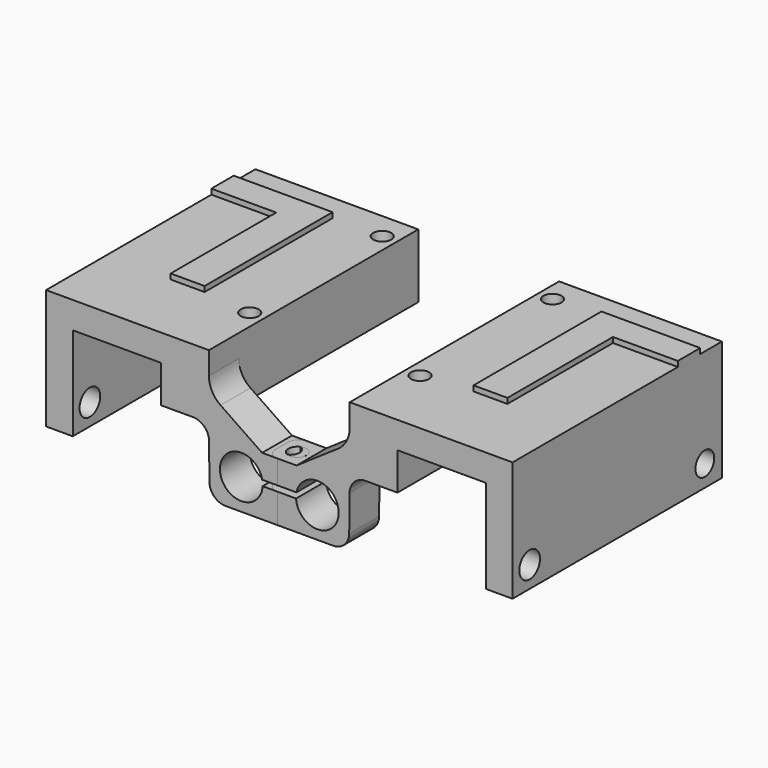
from build123d import *

# Parameters (mm, degrees)
F1_DEPTH      = 7
F2_DEPTH      = 42
F3_R          = 1.7
F3_R_2        = 11
F4_DEPTH      = 12.001
F5_R          = 4
F6_DEPTH      = 10
F7_DEPTH      = 12.001
F8_R          = 1.4
F9_DEPTH      = 10.9920075553
F8_R_2        = 1.7
F10_DEPTH     = 4.4348209087
F11_R         = 5
F12_R         = 3
F13_R         = 3
F14_R         = 2
F15_R         = 2.2
F15_R_2       = 2.4255023423
F16_DEPTH     = 6
F17_TEXT_SIZE = 41.9437823343
F18_DEPTH     = 1


# Not quite as in the source:
# - a feature names something its author has since deleted; it is built from what else it names
# - Text() gives the source's letters only with a copy of the font that has no kerning and outlines rounded to 1/6400 em; it was checked with that copy


with BuildPart() as f1:
    # F0 (on Front) → F1 (new body)
    with BuildSketch(Plane.XZ):
        Polygon((-18.6721007523, 29.8099789735), (-18.6721007523, 7.3259699669), (-13.6721007523, 7.3259699669), (-13.6721007523, 24.8099789735), (2.8778992477, 24.8099789735), (2.8778992477, 17.8099789735), (11.8137966118, 17.8099789735), (11.8137966118, 22.9406704692), (11.8137966118, 29.8099789735), align=None)
        Polygon((21.7801751077, 16.1394868046), (11.8137966118, 22.9406704692), (11.8137966118, 17.8099789735), (11.9440201178, 5.1484792493), (27.3686601057, 5.1484792493), (27.3686601057, 10.6682249423), (20.0360510706, 10.6682249423), (20.0360510706, 11.7046658959), (27.3396428882, 11.7046658959), (27.3396428882, 16.1394868046), align=None)
    extrude(amount=F1_DEPTH)

    # F0 (on Front) → F2 (join)
    with BuildSketch(Plane.XZ):
        Polygon((-18.6721007523, 29.8099789735), (-18.6721007523, 7.3259699669), (-13.6721007523, 7.3259699669), (-13.6721007523, 24.8099789735), (2.8778992477, 24.8099789735), (2.8778992477, 17.8099789735), (11.8137966118, 17.8099789735), (11.8137966118, 22.9406704692), (11.8137966118, 29.8099789735), align=None)
    extrude(amount=-F2_DEPTH)

    # F3 (on face) → F4 (cut, through all)
    with BuildSketch(Plane(origin=(0, 0, 17.8099789735), x_dir=(1, 0, 0), z_dir=(0, 0, -1))):
        with Locations((9.0537966118, -6)):
            Circle(F3_R)
        with Locations((9.0537966118, -37)):
            Circle(F3_R)
        with Locations((24.5537966118, -21.5)):
            Circle(F3_R_2)
    extrude(amount=-F4_DEPTH, mode=Mode.SUBTRACT)

    # F5 (on face) → F6 (cut)
    with BuildSketch(Plane.XZ.offset(7)):
        with Locations((17.8778992477, 10.8989789735)):
            Circle(F5_R)
    extrude(amount=-F6_DEPTH, mode=Mode.SUBTRACT)

    # F3 (on face) → F7 (cut, through all)
    with BuildSketch(Plane(origin=(0, 0, 17.8099789735), x_dir=(1, 0, 0), z_dir=(0, 0, -1))):
        with Locations((9.0537966118, -6)):
            Circle(F3_R)
        with Locations((9.0537966118, -37)):
            Circle(F3_R)
        with Locations((24.5537966118, -21.5)):
            Circle(F3_R_2)
    extrude(amount=-F7_DEPTH, mode=Mode.SUBTRACT)

    # F8 (on face) → F9 (cut, through all)
    with BuildSketch(Plane.XY.offset(16.1394868046)):
        with Locations((24.3396428882, -3.5767070949)):
            Circle(F8_R)
    extrude(amount=-F9_DEPTH, mode=Mode.SUBTRACT)

    # F8 (on face) → F10 (cut, through all)
    with BuildSketch(Plane.XY.offset(16.1394868046)):
        with Locations((24.3396428882, -3.5767070949)):
            Circle(F8_R_2)
        with Locations((24.3396428882, -3.5767070949)):
            Circle(F8_R, mode=Mode.SUBTRACT)
    extrude(amount=-F10_DEPTH, mode=Mode.SUBTRACT)

    # F11
    f11_edges = [f1.edges().sort_by_distance(p)[0] for p in [
        (11.813797, -3.5, 22.94067),
    ]]
    fillet(f11_edges, radius=F11_R)

    # F12
    f12_edges = [f1.edges().sort_by_distance(p)[0] for p in [
        (11.813797, -3.5, 17.809979),
    ]]
    fillet(f12_edges, radius=F12_R)

    # F13
    f13_edges = [f1.edges().sort_by_distance(p)[0] for p in [
        (11.94402, -3.5, 5.148479),
    ]]
    fillet(f13_edges, radius=F13_R)

    # F14
    f14_edges = [f1.edges().sort_by_distance(p)[0] for p in [
        (27.339643, -7, 13.922076),
        (27.36866, -7, 7.908352),
        (27.339643, 0, 13.922076),
        (27.36866, 0, 7.908352),
    ]]
    fillet(f14_edges, radius=F14_R)

    # F15 (on face) → F16 (cut)
    with BuildSketch(Plane(origin=(-18.6721007523, 0, 0), x_dir=(0, -1, 0), z_dir=(-1, 0, 0))):
        with Locations((-38, 11.3259699669)):
            Circle(F15_R)
        with Locations((3, 11.3259699669)):
            Circle(F15_R_2)
    extrude(amount=-F16_DEPTH, mode=Mode.SUBTRACT)

    # F17 (on face) → F18 (join)
    with BuildSketch(Plane.XY.offset(29.8099789735)):
        with Locations(Location((3.5908724648, 36.9253193088), (0, 0, 180))):
            Text('L', F17_TEXT_SIZE, font='Open Sans', font_style=FontStyle.BOLD, text_align=(TextAlign.LEFT, TextAlign.BOTTOM))
    extrude(amount=F18_DEPTH)


with BuildPart() as f19_1:
    # F19: instance of F1
    add(f1.part.mirror(Plane.YZ))


with BuildPart() as f19_1_1:
    # F20: moved
    add(f19_1.part.moved(Location((50, 0, 0))))


solid = Compound([f1.part, f19_1_1.part])
